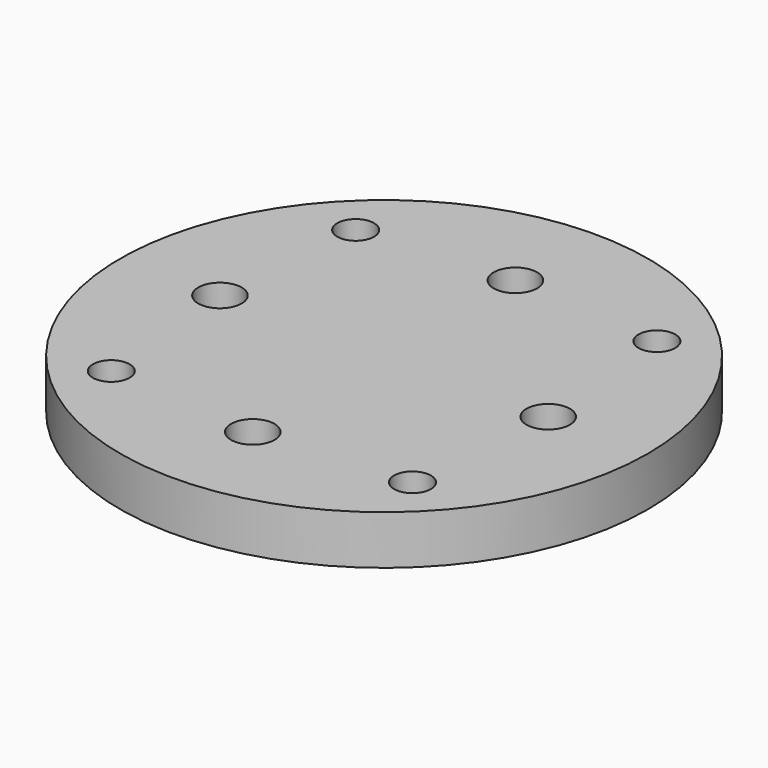
from build123d import *

# Parameters (mm, degrees)
F1_R           = 68.35
F2_DEPTH       = 12.7
F4_D           = 9.525
F4_CSINK_D     = 19.8374
F4_CSINK_ANGLE = 82
F6_D           = 6.6
F6_CBORE_D     = 11.25
F6_CBORE_DEPTH = 6


# Not quite as in the source:
# - a length typed as a fraction of an inch, garbled in the dataset ("3 / 203.2 mm" for 3/8 in), is restored
# - a feature names something its author has since deleted; it is built from what else it names


with BuildPart() as f2:
    # F1 (on Top) → F2 (new body)
    with BuildSketch(Plane.XY):
        Circle(F1_R)
    extrude(amount=F2_DEPTH)

    # F4 (through all)
    with Locations(Plane(origin=(0, 0, 0), x_dir=(1, 0, 0), z_dir=(0, 0, -1))):
        with Locations((-39, -39.5575846078), (39, -39.5575846078), (-39, 39.5575846078), (39, 39.5575846078)):
            CounterSinkHole(F4_D / 2, F4_CSINK_D / 2, counter_sink_angle=F4_CSINK_ANGLE)

    # F6 (through all)
    with Locations(Plane.XY.offset(12.7)):
        with Locations((0, 42.5), (42.5, 0), (0, -42.5), (-42.5, 0)):
            CounterBoreHole(F6_D / 2, F6_CBORE_D / 2, F6_CBORE_DEPTH)


solid = f2.part
